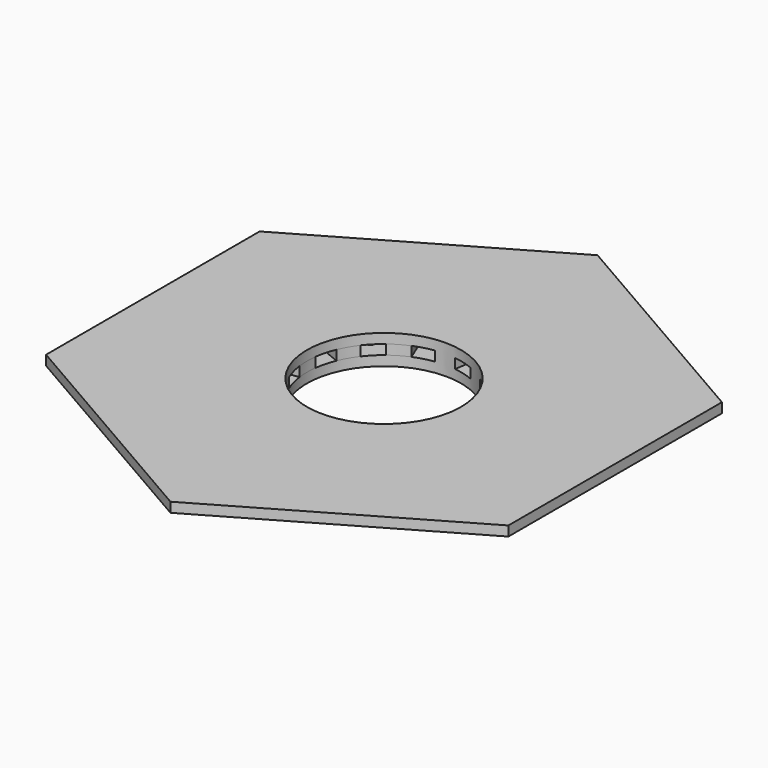
from build123d import *

# Parameters (mm, degrees)
F0_R     = 3.175
F1_DEPTH = 9.525
F3_DEPTH = 9.525
F5_DEPTH = 9.525
F7_DEPTH = 1
F8_R     = 117.5
F8_R_2   = 102.5
F9_DEPTH = 9.525


# Not quite as in the source:
# - a feature names something its author has since deleted; it is built from what else it names


with BuildPart() as f1:
    # F0 (on Top) → F1 (new body)
    with BuildSketch(Plane.XY):
        Polygon((137.2650264998, 79.25), (0, 158.5), (-137.2650264998, 79.25), (-137.2650264998, -79.25), (0, -158.5), (137.2650264998, -79.25), align=None)
        with Locations((-88.3883476483, -88.3883476483)):
            Circle(F0_R, mode=Mode.SUBTRACT)
        with Locations((-32.3523806378, -120.7407282861)):
            Circle(F0_R, mode=Mode.SUBTRACT)
        with Locations((-24.5878092847, -91.7629534975)):
            Circle(F0_R, mode=Mode.SUBTRACT)
        with Locations((-120.7407282861, -32.3523806378)):
            Circle(F0_R, mode=Mode.SUBTRACT)
        with Locations((-91.7629534975, -24.5878092847)):
            Circle(F0_R, mode=Mode.SUBTRACT)
        with Locations((-67.1751442127, -67.1751442127)):
            Circle(F0_R, mode=Mode.SUBTRACT)
        with Locations((32.3523806378, -120.7407282861)):
            Circle(F0_R, mode=Mode.SUBTRACT)
        with Locations((24.5878092847, -91.7629534975)):
            Circle(F0_R, mode=Mode.SUBTRACT)
        with Locations((88.3883476483, -88.3883476483)):
            Circle(F0_R, mode=Mode.SUBTRACT)
        with Locations((67.1751442127, -67.1751442127)):
            Circle(F0_R, mode=Mode.SUBTRACT)
        with Locations((91.7629534975, -24.5878092847)):
            Circle(F0_R, mode=Mode.SUBTRACT)
        with Locations((120.7407282861, -32.3523806378)):
            Circle(F0_R, mode=Mode.SUBTRACT)
        with Locations((-120.7407282861, 32.3523806378)):
            Circle(F0_R, mode=Mode.SUBTRACT)
        with Locations((-91.7629534975, 24.5878092847)):
            Circle(F0_R, mode=Mode.SUBTRACT)
        with Locations((-67.1751442127, 67.1751442127)):
            Circle(F0_R, mode=Mode.SUBTRACT)
        with Locations((-88.3883476483, 88.3883476483)):
            Circle(F0_R, mode=Mode.SUBTRACT)
        with Locations((-24.5878092847, 91.7629534975)):
            Circle(F0_R, mode=Mode.SUBTRACT)
        with Locations((-32.3523806378, 120.7407282861)):
            Circle(F0_R, mode=Mode.SUBTRACT)
        with BuildLine():
            ThreePointArc((75, 0), (-53.033008589, -53.033008589), (0, 75))
            ThreePointArc((0, 75), (9.7894644165, 74.358364603), (19.4114283827, 72.4444369717))
            ThreePointArc((19.4114283827, 72.4444369717), (59.5015005218, 45.6571071757), (75, 0))
        make_face(mode=Mode.SUBTRACT)
        with Locations((67.1751442127, 67.1751442127)):
            Circle(F0_R, mode=Mode.SUBTRACT)
        with Locations((91.7629534975, 24.5878092847)):
            Circle(F0_R, mode=Mode.SUBTRACT)
        with Locations((120.7407282861, 32.3523806378)):
            Circle(F0_R, mode=Mode.SUBTRACT)
        with BuildLine():
            ThreePointArc((27.7628092847, 91.7629534975), (26.5206268218, 89.244056642), (23.7660588165, 88.696138999))
            ThreePointArc((23.7660588165, 88.696138999), (21.5209947863, 92.5847039657), (25.4095597529, 94.8297679959))
            ThreePointArc((25.4095597529, 94.8297679959), (27.1067061402, 93.6957710346), (27.7628092847, 91.7629534975))
        make_face(mode=Mode.SUBTRACT)
        with BuildLine():
            ThreePointArc((35.5273806378, 120.7407282861), (34.2851981749, 118.2218314307), (31.5306301696, 117.6739137877))
            ThreePointArc((31.5306301696, 117.6739137877), (30.4195631007, 123.2596251416), (35.5273806378, 120.7407282861))
        make_face(mode=Mode.SUBTRACT)
        with Locations((88.3883476483, 88.3883476483)):
            Circle(F0_R, mode=Mode.SUBTRACT)
    extrude(amount=F1_DEPTH)

    # F2 (on face) → F3 (join)
    with BuildSketch(Plane.XY.offset(9.525)):
        Polygon((52.9823225992, 127.9106417851), (84.2827039006, 109.8393582149), (89.1948191597, 116.2409514549), (56.0702073402, 135.3654550057), align=None)
        Polygon((-20.523120282, 155.8885752876), (-19.3928760228, 147.3035178079), (0, 158.5), (19.3928760228, 147.3035178079), (20.523120282, 155.8885752876), (0, 167.737604307), align=None)
        Polygon((-137.2650264998, -18.0712835701), (-137.2650264998, 18.0712835701), (-145.2650264998, 19.1245035508), (-145.2650264998, -19.1245035508), align=None)
        Polygon((-137.2650264998, -79.25), (-137.2650264998, -56.8570356157), (-145.2650264998, -60.1707441147), (-145.2650264998, -83.8688021535), (-124.7419062179, -95.7178311729), (-117.872150477, -90.4464821921), align=None)
        Polygon((0, -167.737604307), (20.523120282, -155.8885752876), (19.3928760228, -147.3035178079), (0, -158.5), (-19.3928760228, -147.3035178079), (-20.523120282, -155.8885752876), align=None)
        Polygon((56.0702073402, -135.3654550057), (89.1948191597, -116.2409514549), (84.2827039006, -109.8393582149), (52.9823225992, -127.9106417851), align=None)
        Polygon((124.7419062179, -95.7178311729), (145.2650264998, -83.8688021535), (145.2650264998, -60.1707441147), (137.2650264998, -56.8570356157), (137.2650264998, -79.25), (117.872150477, -90.4464821921), align=None)
        Polygon((137.2650264998, 56.8570356157), (145.2650264998, 60.1707441147), (145.2650264998, 83.8688021535), (124.7419062179, 95.7178311729), (117.872150477, 90.4464821921), (137.2650264998, 79.25), align=None)
        Polygon((-137.2650264998, 79.25), (-117.872150477, 90.4464821921), (-124.7419062179, 95.7178311729), (-145.2650264998, 83.8688021535), (-145.2650264998, 60.1707441147), (-137.2650264998, 56.8570356157), align=None)
        with BuildLine():
            ThreePointArc((-69.2909649383, 28.7012574274), (-64.9519052838, 37.5), (-59.5015005218, 45.6571071757))
            Line((-59.5015005218, 45.6571071757), (-117.872150477, 90.4464821921))
            Line((-117.872150477, 90.4464821921), (-137.2650264998, 79.25))
            Line((-137.2650264998, 79.25), (-137.2650264998, 56.8570356157))
            Line((-137.2650264998, 56.8570356157), (-69.2909649383, 28.7012574274))
        make_face()
        with BuildLine():
            ThreePointArc((28.7012574274, 69.2909649383), (37.5, 64.9519052838), (45.6571071757, 59.5015005218))
            Line((45.6571071757, 59.5015005218), (84.2827039006, 109.8393582149))
            Line((84.2827039006, 109.8393582149), (52.9823225992, 127.9106417851))
            Line((52.9823225992, 127.9106417851), (28.7012574274, 69.2909649383))
        make_face()
        with BuildLine():
            ThreePointArc((59.5015005218, 45.6571071757), (64.9519052838, 37.5), (69.2909649383, 28.7012574274))
            Line((69.2909649383, 28.7012574274), (137.2650264998, 56.8570356157))
            Line((137.2650264998, 56.8570356157), (137.2650264998, 79.25))
            Line((137.2650264998, 79.25), (117.872150477, 90.4464821921))
            Line((117.872150477, 90.4464821921), (59.5015005218, 45.6571071757))
        make_face()
        with BuildLine():
            Line((59.5015005218, -45.6571071757), (117.872150477, -90.4464821921))
            Line((117.872150477, -90.4464821921), (137.2650264998, -79.25))
            Line((137.2650264998, -79.25), (137.2650264998, -56.8570356157))
            Line((137.2650264998, -56.8570356157), (69.2909649383, -28.7012574274))
            ThreePointArc((69.2909649383, -28.7012574274), (64.9519052838, -37.5), (59.5015005218, -45.6571071757))
        make_face()
        with BuildLine():
            Line((52.9823225992, -127.9106417851), (84.2827039006, -109.8393582149))
            Line((84.2827039006, -109.8393582149), (45.6571071757, -59.5015005218))
            ThreePointArc((45.6571071757, -59.5015005218), (37.5, -64.9519052838), (28.7012574274, -69.2909649383))
            Line((28.7012574274, -69.2909649383), (52.9823225992, -127.9106417851))
        make_face()
        with BuildLine():
            Line((0, -158.5), (19.3928760228, -147.3035178079))
            Line((19.3928760228, -147.3035178079), (9.7894644165, -74.358364603))
            ThreePointArc((9.7894644165, -74.358364603), (0, -75), (-9.7894644165, -74.358364603))
            Line((-9.7894644165, -74.358364603), (-19.3928760228, -147.3035178079))
            Line((-19.3928760228, -147.3035178079), (0, -158.5))
        make_face()
        with BuildLine():
            ThreePointArc((-59.5015005218, -45.6571071757), (-64.9519052838, -37.5), (-69.2909649383, -28.7012574274))
            Line((-69.2909649383, -28.7012574274), (-137.2650264998, -56.8570356157))
            Line((-137.2650264998, -56.8570356157), (-137.2650264998, -79.25))
            Line((-137.2650264998, -79.25), (-117.872150477, -90.4464821921))
            Line((-117.872150477, -90.4464821921), (-59.5015005218, -45.6571071757))
        make_face()
        with BuildLine():
            ThreePointArc((-74.358364603, -9.7894644165), (-75, 0), (-74.358364603, 9.7894644165))
            Line((-74.358364603, 9.7894644165), (-137.2650264998, 18.0712835701))
            Line((-137.2650264998, 18.0712835701), (-137.2650264998, -18.0712835701))
            Line((-137.2650264998, -18.0712835701), (-74.358364603, -9.7894644165))
        make_face()
        with BuildLine():
            Line((75, 0), (137.2650264998, 0))
            Line((137.2650264998, 0), (137.2650264998, 18.0712835701))
            Line((137.2650264998, 18.0712835701), (74.358364603, 9.7894644165))
            ThreePointArc((74.358364603, 9.7894644165), (74.8394192429, 4.9052346923), (75, 0))
        make_face()
        with BuildLine():
            Line((74.358364603, -9.7894644165), (137.2650264998, -18.0712835701))
            Line((137.2650264998, -18.0712835701), (137.2650264998, 0))
            Line((137.2650264998, 0), (75, 0))
            ThreePointArc((75, 0), (74.8394192429, -4.9052346923), (74.358364603, -9.7894644165))
        make_face()
        Polygon((137.2650264998, 0), (145.2650264998, 0), (145.2650264998, 19.1245035508), (137.2650264998, 18.0712835701), align=None)
        Polygon((137.2650264998, -18.0712835701), (145.2650264998, -19.1245035508), (145.2650264998, 0), (137.2650264998, 0), align=None)
        Polygon((-52.9823225992, -127.9106417851), (-84.2827039006, -109.8393582149), (-89.1948191597, -116.2409514549), (-56.0702073402, -135.3654550057), align=None)
        with BuildLine():
            ThreePointArc((-28.7012574274, -69.2909649383), (-37.5, -64.9519052838), (-45.6571071757, -59.5015005218))
            Line((-45.6571071757, -59.5015005218), (-84.2827039006, -109.8393582149))
            Line((-84.2827039006, -109.8393582149), (-52.9823225992, -127.9106417851))
            Line((-52.9823225992, -127.9106417851), (-28.7012574274, -69.2909649383))
        make_face()
        Polygon((-84.2827039006, 109.8393582149), (-52.9823225992, 127.9106417851), (-56.0702073402, 135.3654550057), (-89.1948191597, 116.2409514549), align=None)
        with BuildLine():
            ThreePointArc((-45.6571071757, 59.5015005218), (-37.5, 64.9519052838), (-28.7012574274, 69.2909649383))
            Line((-28.7012574274, 69.2909649383), (-52.9823225992, 127.9106417851))
            Line((-52.9823225992, 127.9106417851), (-84.2827039006, 109.8393582149))
            Line((-84.2827039006, 109.8393582149), (-45.6571071757, 59.5015005218))
        make_face()
        with BuildLine():
            Line((-19.3928760228, 147.3035178079), (-9.7894644165, 74.358364603))
            ThreePointArc((-9.7894644165, 74.358364603), (0, 75), (9.7894644165, 74.358364603))
            Line((9.7894644165, 74.358364603), (19.3928760228, 147.3035178079))
            Line((19.3928760228, 147.3035178079), (0, 158.5))
            Line((0, 158.5), (-19.3928760228, 147.3035178079))
        make_face()
    extrude(amount=F3_DEPTH)

    # F4 (on face) → F5 (join)
    with BuildSketch(Plane.XY.offset(19.05)):
        Polygon((225, 129.9038105677), (0, 259.8076211353), (-225, 129.9038105677), (-225, -129.9038105677), (0, -259.8076211353), (225, -129.9038105677), align=None)
        with BuildLine():
            ThreePointArc((75, 0), (-45.6571071757, -59.5015005218), (-19.4114283827, 72.4444369717))
            ThreePointArc((-19.4114283827, 72.4444369717), (-14.6317741512, 73.5588960302), (-9.7894644165, 74.358364603))
            Line((-9.7894644165, 74.358364603), (-20.523120282, 155.8885752876))
            Line((-20.523120282, 155.8885752876), (0, 167.737604307))
            Line((0, 167.737604307), (20.523120282, 155.8885752876))
            Line((20.523120282, 155.8885752876), (9.7894644165, 74.358364603))
            ThreePointArc((9.7894644165, 74.358364603), (56.3879855609, 49.4509361325), (75, 0))
        make_face(mode=Mode.SUBTRACT)
        with BuildLine():
            ThreePointArc((-9.7894644165, 74.358364603), (-4.9052346923, 74.8394192429), (0, 75))
            ThreePointArc((0, 75), (4.9052346923, 74.8394192429), (9.7894644165, 74.358364603))
            Line((9.7894644165, 74.358364603), (20.523120282, 155.8885752876))
            Line((20.523120282, 155.8885752876), (0, 167.737604307))
            Line((0, 167.737604307), (-20.523120282, 155.8885752876))
            Line((-20.523120282, 155.8885752876), (-9.7894644165, 74.358364603))
        make_face()
    extrude(amount=F5_DEPTH)

    # F6 (on face) → F7 (cut)
    with BuildSketch(Plane(origin=(0, 0, 19.05), x_dir=(1, 0, 0), z_dir=(0, 0, -1))):
        Polygon((20.1049319239, 113.6696604743), (17.5167414729, 104.0104022114), (27.1759997358, 101.4222117604), (29.7641901868, 111.0814700232), align=None)
        Polygon((31.7517889535, 157.1363226573), (41.4110472164, 154.5481322063), (51.0703054793, 151.9599417552), (53.6584959303, 161.6192000181), (34.3399794045, 166.7955809202), align=None)
        Polygon((29.7641901868, 111.0814700232), (27.1759997358, 101.4222117604), (36.8352579987, 98.8340213093), (39.4234484497, 108.4932795722), align=None)
        Polygon((-51.0703054793, 151.9599417552), (-31.7517889535, 157.1363226573), (-34.3399794045, 166.7955809202), (-53.6584959303, 161.6192000181), align=None)
        Polygon((-39.4234484497, 108.4932795722), (-36.8352579987, 98.8340213093), (-27.1759997358, 101.4222117604), (-29.7641901868, 111.0814700232), align=None)
        Polygon((-29.7641901868, 111.0814700232), (-27.1759997358, 101.4222117604), (-17.5167414729, 104.0104022114), (-20.1049319239, 113.6696604743), align=None)
        Polygon((-120.2081528017, 106.066017178), (-106.066017178, 120.2081528017), (-113.1370849898, 127.2792206136), (-127.2792206136, 113.1370849898), align=None)
        Polygon((-88.3883476483, 74.2462120246), (-81.3172798365, 67.1751442127), (-74.2462120246, 74.2462120246), (-81.3172798365, 81.3172798365), align=None)
        Polygon((-81.3172798365, 81.3172798365), (-74.2462120246, 74.2462120246), (-67.1751442127, 81.3172798365), (-74.2462120246, 88.3883476483), align=None)
        Polygon((-157.1363226573, 31.7517889535), (-151.9599417552, 51.0703054793), (-161.6192000181, 53.6584959303), (-166.7955809202, 34.3399794045), align=None)
        Polygon((-113.6696604743, 20.1049319239), (-104.0104022114, 17.5167414729), (-101.4222117604, 27.1759997358), (-111.0814700232, 29.7641901868), align=None)
        Polygon((-111.0814700232, 29.7641901868), (-101.4222117604, 27.1759997358), (-98.8340213093, 36.8352579987), (-108.4932795722, 39.4234484497), align=None)
        Polygon((-151.9599417552, -51.0703054793), (-157.1363226573, -31.7517889535), (-166.7955809202, -34.3399794045), (-161.6192000181, -53.6584959303), align=None)
        Polygon((-108.4932795722, -39.4234484497), (-98.8340213093, -36.8352579987), (-101.4222117604, -27.1759997358), (-111.0814700232, -29.7641901868), align=None)
        Polygon((-111.0814700232, -29.7641901868), (-101.4222117604, -27.1759997358), (-104.0104022114, -17.5167414729), (-113.6696604743, -20.1049319239), align=None)
        Polygon((-106.066017178, -120.2081528017), (-120.2081528017, -106.066017178), (-127.2792206136, -113.1370849898), (-113.1370849898, -127.2792206136), align=None)
        Polygon((-74.2462120246, -88.3883476483), (-67.1751442127, -81.3172798365), (-74.2462120246, -74.2462120246), (-81.3172798365, -81.3172798365), align=None)
        Polygon((-81.3172798365, -81.3172798365), (-74.2462120246, -74.2462120246), (-81.3172798365, -67.1751442127), (-88.3883476483, -74.2462120246), align=None)
        Polygon((-31.7517889535, -157.1363226573), (-51.0703054793, -151.9599417552), (-53.6584959303, -161.6192000181), (-34.3399794045, -166.7955809202), align=None)
        Polygon((-20.1049319239, -113.6696604743), (-17.5167414729, -104.0104022114), (-27.1759997358, -101.4222117604), (-29.7641901868, -111.0814700232), align=None)
        Polygon((-29.7641901868, -111.0814700232), (-27.1759997358, -101.4222117604), (-36.8352579987, -98.8340213093), (-39.4234484497, -108.4932795722), align=None)
        Polygon((51.0703054793, -151.9599417552), (31.7517889535, -157.1363226573), (34.3399794045, -166.7955809202), (53.6584959303, -161.6192000181), align=None)
        Polygon((39.4234484497, -108.4932795722), (36.8352579987, -98.8340213093), (27.1759997358, -101.4222117604), (29.7641901868, -111.0814700232), align=None)
        Polygon((29.7641901868, -111.0814700232), (27.1759997358, -101.4222117604), (17.5167414729, -104.0104022114), (20.1049319239, -113.6696604743), align=None)
        Polygon((120.2081528017, -106.066017178), (106.066017178, -120.2081528017), (113.1370849898, -127.2792206136), (127.2792206136, -113.1370849898), align=None)
        Polygon((88.3883476483, -74.2462120246), (81.3172798365, -67.1751442127), (74.2462120246, -74.2462120246), (81.3172798365, -81.3172798365), align=None)
        Polygon((81.3172798365, -81.3172798365), (74.2462120246, -74.2462120246), (67.1751442127, -81.3172798365), (74.2462120246, -88.3883476483), align=None)
        Polygon((157.1363226573, -31.7517889535), (151.9599417552, -51.0703054793), (161.6192000181, -53.6584959303), (166.7955809202, -34.3399794045), align=None)
        Polygon((113.6696604743, -20.1049319239), (104.0104022114, -17.5167414729), (101.4222117604, -27.1759997358), (111.0814700232, -29.7641901868), align=None)
        Polygon((111.0814700232, -29.7641901868), (101.4222117604, -27.1759997358), (98.8340213093, -36.8352579987), (108.4932795722, -39.4234484497), align=None)
        Polygon((151.9599417552, 51.0703054793), (157.1363226573, 31.7517889535), (166.7955809202, 34.3399794045), (161.6192000181, 53.6584959303), align=None)
        Polygon((108.4932795722, 39.4234484497), (98.8340213093, 36.8352579987), (101.4222117604, 27.1759997358), (111.0814700232, 29.7641901868), align=None)
        Polygon((111.0814700232, 29.7641901868), (101.4222117604, 27.1759997358), (104.0104022114, 17.5167414729), (113.6696604743, 20.1049319239), align=None)
        Polygon((106.066017178, 120.2081528017), (120.2081528017, 106.066017178), (127.2792206136, 113.1370849898), (113.1370849898, 127.2792206136), align=None)
        Polygon((74.2462120246, 88.3883476483), (67.1751442127, 81.3172798365), (74.2462120246, 74.2462120246), (81.3172798365, 81.3172798365), align=None)
        Polygon((81.3172798365, 81.3172798365), (74.2462120246, 74.2462120246), (81.3172798365, 67.1751442127), (88.3883476483, 74.2462120246), align=None)
    extrude(amount=-F7_DEPTH, mode=Mode.SUBTRACT)

    # F8 (on face) → F9 (cut)
    with BuildSketch(Plane(origin=(0, 0, 0), x_dir=(1, 0, 0), z_dir=(0, 0, -1))):
        Circle(F8_R)
        Circle(F8_R_2, mode=Mode.SUBTRACT)
    extrude(amount=-F9_DEPTH, mode=Mode.SUBTRACT)


solid = f1.part
